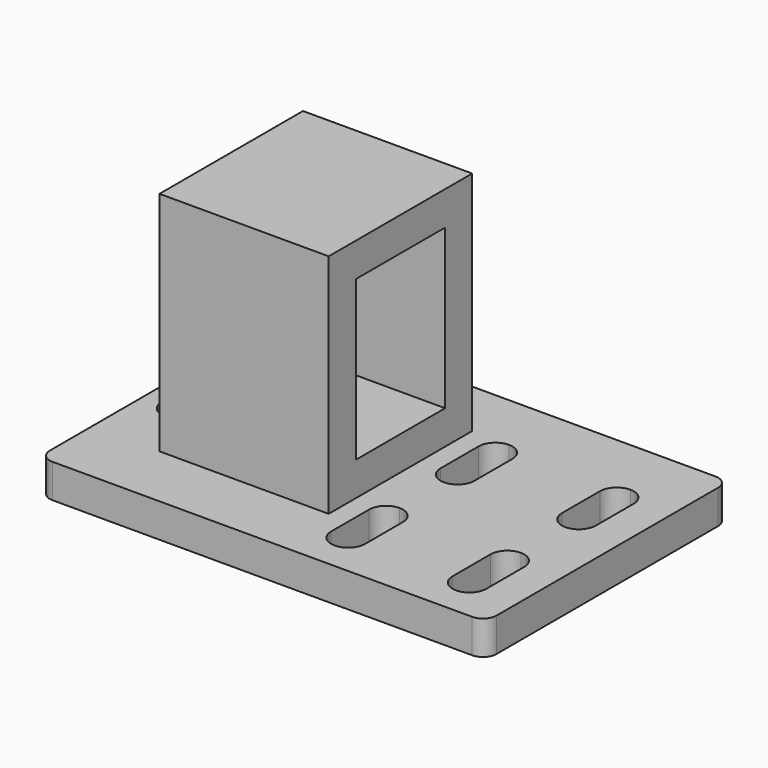
from build123d import *

# Parameters (mm, degrees)
F0_W          = 26.5
F0_H          = 33.5
F1_DEPTH      = 25
F2_W          = 16.5
F2_H          = 23.5
F3_DEPTH      = 20
F4_R          = 2.5
F5_DEPTH      = 25.001
F7_DEPTH      = 31
F7_DEPTH_BACK = 35
F8_R          = 2
F10_DEPTH     = 5


# Not quite as in the source:
# - a feature names something its author has since deleted; it is built from what else it names


with BuildPart() as f1:
    # F0 (on Right) → F1 (new body)
    with BuildSketch(Plane.YZ):
        with Locations((8.25, 11.75)):
            Rectangle(F0_W, F0_H)
    extrude(amount=F1_DEPTH)

    # F2 (on face) → F3 (cut)
    with BuildSketch(Plane.YZ.offset(25)):
        with Locations((8.25, 11.75)):
            Rectangle(F2_W, F2_H)
    extrude(amount=-F3_DEPTH, mode=Mode.SUBTRACT)

    # F4 (on face) → F5 (cut, through all)
    with BuildSketch(Plane(origin=(0, 0, 0), x_dir=(0, -1, 0), z_dir=(-1, 0, 0))):
        with Locations((-8.25, 11.75)):
            Circle(F4_R)
    extrude(amount=-F5_DEPTH, mode=Mode.SUBTRACT)

    # F6 (on face) → F7 (join, two sides)
    with BuildSketch(Plane.YZ.offset(25)) as f7_sk:
        Polygon((-5, -5), (-14.75, -5), (-14.75, -10), (30.18, -10), (30.18, -5), (21.5, -5), align=None)
    extrude(amount=F7_DEPTH)
    extrude(f7_sk.sketch, amount=-F7_DEPTH_BACK)

    # F8
    f8_edges = [f1.edges().sort_by_distance(p)[0] for p in [
        (56, -14.75, -7.5),
        (56, 30.18, -7.5),
        (-10, -14.75, -7.5),
        (-10, 30.18, -7.5),
    ]]
    fillet(f8_edges, radius=F8_R)

    # F9 (on face) → F10 (cut, through all)
    with BuildSketch(Plane.XY.offset(-5)):
        with BuildLine():
            ThreePointArc((30.47, 21.46), (28.702233047, 20.727766953), (27.97, 18.96))
            Line((27.97, 18.96), (27.97, 11.96))
            ThreePointArc((27.97, 11.96), (28.702233047, 10.192233047), (30.47, 9.46))
            ThreePointArc((30.47, 9.46), (32.237766953, 10.192233047), (32.97, 11.96))
            Line((32.97, 11.96), (32.97, 18.96))
            ThreePointArc((32.97, 18.96), (32.237766953, 20.727766953), (30.47, 21.46))
        make_face()
        with BuildLine():
            ThreePointArc((30.47, 1.25), (28.702233047, 0.517766953), (27.97, -1.25))
            Line((27.97, -1.25), (27.97, -8.25))
            ThreePointArc((27.97, -8.25), (28.702233047, -10.017766953), (30.47, -10.75))
            ThreePointArc((30.47, -10.75), (32.237766953, -10.017766953), (32.97, -8.25))
            Line((32.97, -8.25), (32.97, -1.25))
            ThreePointArc((32.97, -1.25), (32.237766953, 0.517766953), (30.47, 1.25))
        make_face()
        with BuildLine():
            ThreePointArc((48.4, 21.46), (46.632233047, 20.727766953), (45.9, 18.96))
            Line((45.9, 18.96), (45.9, 11.96))
            ThreePointArc((45.9, 11.96), (46.632233047, 10.192233047), (48.4, 9.46))
            ThreePointArc((48.4, 9.46), (50.167766953, 10.192233047), (50.9, 11.96))
            Line((50.9, 11.96), (50.9, 18.96))
            ThreePointArc((50.9, 18.96), (50.167766953, 20.727766953), (48.4, 21.46))
        make_face()
        with BuildLine():
            ThreePointArc((48.4, 1.25), (46.632233047, 0.517766953), (45.9, -1.25))
            Line((45.9, -1.25), (45.9, -8.25))
            ThreePointArc((45.9, -8.25), (46.632233047, -10.017766953), (48.4, -10.75))
            ThreePointArc((48.4, -10.75), (50.167766953, -10.017766953), (50.9, -8.25))
            Line((50.9, -8.25), (50.9, -1.25))
            ThreePointArc((50.9, -1.25), (50.167766953, 0.517766953), (48.4, 1.25))
        make_face()
        with BuildLine():
            ThreePointArc((-5, 14.25), (-6.767766953, 13.517766953), (-7.5, 11.75))
            Line((-7.5, 11.75), (-7.5, 4.75))
            ThreePointArc((-7.5, 4.75), (-6.767766953, 2.982233047), (-5, 2.25))
            ThreePointArc((-5, 2.25), (-3.232233047, 2.982233047), (-2.5, 4.75))
            Line((-2.5, 4.75), (-2.5, 11.75))
            ThreePointArc((-2.5, 11.75), (-3.232233047, 13.517766953), (-5, 14.25))
        make_face()
    extrude(amount=-F10_DEPTH, mode=Mode.SUBTRACT)


solid = f1.part
